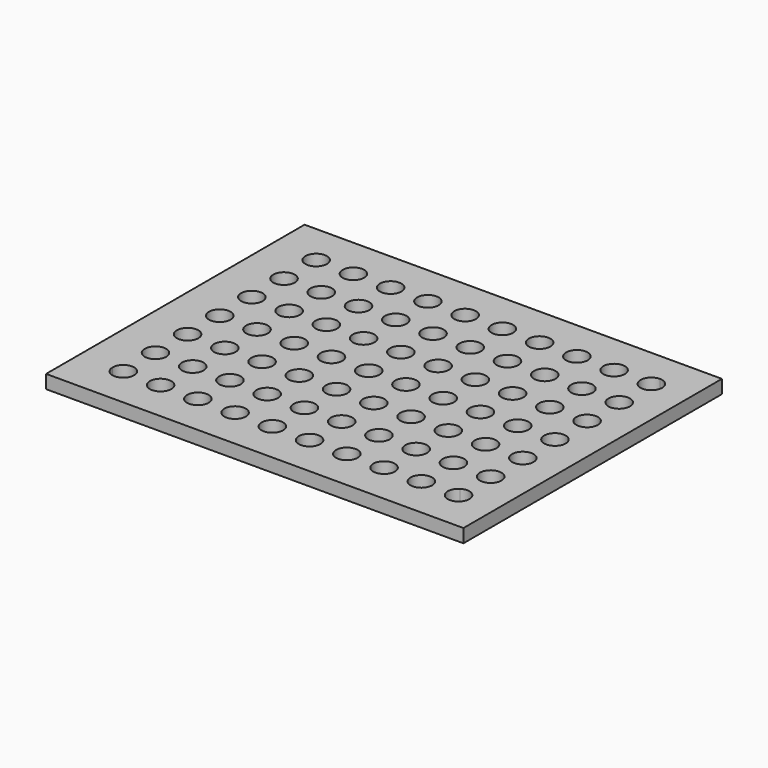
from build123d import *

# Parameters (mm, degrees)
F0_W     = 620
F0_H     = 480
F0_R     = 16
F1_DEPTH = 20


# Not quite as in the source:
# - ends of sketch curves that miss each other by under 0.0002 mm in the source are joined


with BuildPart() as f1:
    # F0 (on Top) → F1 (new body)
    with BuildSketch(Plane.XY):
        Rectangle(F0_W, F0_H)
        with BuildLine():
            ThreePointArc((-228, -179), (-228.000003125, -179.0099999941), (-228.0000125, -179.0199999844))
            ThreePointArc((-228.0000125, -179.0199999844), (-244.0050000002, -195.0199992187), (-259.999996875, -179.01))
            ThreePointArc((-259.999996875, -179.01), (-244.0050000002, -163.0000007813), (-228, -179))
        make_face(mode=Mode.SUBTRACT)
        with Locations((-188.67, -179.02)):
            Circle(F0_R, mode=Mode.SUBTRACT)
        with Locations((-133.34, -179.02)):
            Circle(F0_R, mode=Mode.SUBTRACT)
        with Locations((-78.01, -179.02)):
            Circle(F0_R, mode=Mode.SUBTRACT)
        with Locations((-22.68, -179.02)):
            Circle(F0_R, mode=Mode.SUBTRACT)
        with Locations((-244, -119.35)):
            Circle(F0_R, mode=Mode.SUBTRACT)
        with Locations((-188.67, -119.35)):
            Circle(F0_R, mode=Mode.SUBTRACT)
        with Locations((-244, -59.68)):
            Circle(F0_R, mode=Mode.SUBTRACT)
        with Locations((-244, -0.01)):
            Circle(F0_R, mode=Mode.SUBTRACT)
        with Locations((-188.67, -59.68)):
            Circle(F0_R, mode=Mode.SUBTRACT)
        with Locations((-188.67, -0.01)):
            Circle(F0_R, mode=Mode.SUBTRACT)
        with Locations((-133.34, -119.35)):
            Circle(F0_R, mode=Mode.SUBTRACT)
        with Locations((-78.01, -119.35)):
            Circle(F0_R, mode=Mode.SUBTRACT)
        with Locations((-22.68, -119.35)):
            Circle(F0_R, mode=Mode.SUBTRACT)
        with Locations((-133.34, -59.68)):
            Circle(F0_R, mode=Mode.SUBTRACT)
        with Locations((-78.01, -59.68)):
            Circle(F0_R, mode=Mode.SUBTRACT)
        with Locations((-133.34, -0.01)):
            Circle(F0_R, mode=Mode.SUBTRACT)
        with Locations((-78.01, -0.01)):
            Circle(F0_R, mode=Mode.SUBTRACT)
        with Locations((-22.68, -59.68)):
            Circle(F0_R, mode=Mode.SUBTRACT)
        with Locations((-22.68, -0.01)):
            Circle(F0_R, mode=Mode.SUBTRACT)
        with Locations((32.65, -179.02)):
            Circle(F0_R, mode=Mode.SUBTRACT)
        with Locations((87.98, -179.02)):
            Circle(F0_R, mode=Mode.SUBTRACT)
        with Locations((143.31, -179.02)):
            Circle(F0_R, mode=Mode.SUBTRACT)
        with Locations((198.64, -179.02)):
            Circle(F0_R, mode=Mode.SUBTRACT)
        with BuildLine():
            ThreePointArc((245.1098024941, -165.6972037411), (261.5417783017, -164.8889553878), (270, -179))
            ThreePointArc((270, -179), (268.1025380711, -186.5576729191), (262.8601975059, -192.3227962589))
            ThreePointArc((262.8601975059, -192.3227962589), (240.6571952906, -187.8952031396), (245.1098024941, -165.6972037411))
        make_face(mode=Mode.SUBTRACT)
        with Locations((32.65, -119.35)):
            Circle(F0_R, mode=Mode.SUBTRACT)
        with Locations((87.98, -119.35)):
            Circle(F0_R, mode=Mode.SUBTRACT)
        with Locations((143.31, -119.35)):
            Circle(F0_R, mode=Mode.SUBTRACT)
        with Locations((32.65, -59.68)):
            Circle(F0_R, mode=Mode.SUBTRACT)
        with Locations((32.65, -0.01)):
            Circle(F0_R, mode=Mode.SUBTRACT)
        with Locations((87.98, -59.68)):
            Circle(F0_R, mode=Mode.SUBTRACT)
        with Locations((143.31, -59.68)):
            Circle(F0_R, mode=Mode.SUBTRACT)
        with Locations((87.98, -0.01)):
            Circle(F0_R, mode=Mode.SUBTRACT)
        with Locations((143.31, -0.01)):
            Circle(F0_R, mode=Mode.SUBTRACT)
        with Locations((198.64, -119.35)):
            Circle(F0_R, mode=Mode.SUBTRACT)
        with Locations((253.97, -119.35)):
            Circle(F0_R, mode=Mode.SUBTRACT)
        with Locations((198.64, -59.68)):
            Circle(F0_R, mode=Mode.SUBTRACT)
        with Locations((198.64, -0.01)):
            Circle(F0_R, mode=Mode.SUBTRACT)
        with Locations((253.97, -59.68)):
            Circle(F0_R, mode=Mode.SUBTRACT)
        with Locations((253.97, -0.01)):
            Circle(F0_R, mode=Mode.SUBTRACT)
        with Locations((-244, 59.66)):
            Circle(F0_R, mode=Mode.SUBTRACT)
        with Locations((-188.67, 59.66)):
            Circle(F0_R, mode=Mode.SUBTRACT)
        with Locations((-244, 119.33)):
            Circle(F0_R, mode=Mode.SUBTRACT)
        with Locations((-188.67, 119.33)):
            Circle(F0_R, mode=Mode.SUBTRACT)
        with Locations((-133.34, 59.66)):
            Circle(F0_R, mode=Mode.SUBTRACT)
        with Locations((-78.01, 59.66)):
            Circle(F0_R, mode=Mode.SUBTRACT)
        with Locations((-22.68, 59.66)):
            Circle(F0_R, mode=Mode.SUBTRACT)
        with Locations((-133.34, 119.33)):
            Circle(F0_R, mode=Mode.SUBTRACT)
        with Locations((-78.01, 119.33)):
            Circle(F0_R, mode=Mode.SUBTRACT)
        with Locations((-22.68, 119.33)):
            Circle(F0_R, mode=Mode.SUBTRACT)
        with Locations((-244, 179)):
            Circle(F0_R, mode=Mode.SUBTRACT)
        with Locations((-188.67, 179)):
            Circle(F0_R, mode=Mode.SUBTRACT)
        with Locations((-133.34, 179)):
            Circle(F0_R, mode=Mode.SUBTRACT)
        with Locations((-78.01, 179)):
            Circle(F0_R, mode=Mode.SUBTRACT)
        with Locations((-22.68, 179)):
            Circle(F0_R, mode=Mode.SUBTRACT)
        with Locations((32.65, 59.66)):
            Circle(F0_R, mode=Mode.SUBTRACT)
        with Locations((87.98, 59.66)):
            Circle(F0_R, mode=Mode.SUBTRACT)
        with Locations((143.31, 59.66)):
            Circle(F0_R, mode=Mode.SUBTRACT)
        with Locations((32.65, 119.33)):
            Circle(F0_R, mode=Mode.SUBTRACT)
        with Locations((87.98, 119.33)):
            Circle(F0_R, mode=Mode.SUBTRACT)
        with Locations((143.31, 119.33)):
            Circle(F0_R, mode=Mode.SUBTRACT)
        with Locations((198.64, 59.66)):
            Circle(F0_R, mode=Mode.SUBTRACT)
        with Locations((253.97, 59.66)):
            Circle(F0_R, mode=Mode.SUBTRACT)
        with Locations((198.64, 119.33)):
            Circle(F0_R, mode=Mode.SUBTRACT)
        with Locations((253.97, 119.33)):
            Circle(F0_R, mode=Mode.SUBTRACT)
        with Locations((32.65, 179)):
            Circle(F0_R, mode=Mode.SUBTRACT)
        with Locations((87.98, 179)):
            Circle(F0_R, mode=Mode.SUBTRACT)
        with Locations((143.31, 179)):
            Circle(F0_R, mode=Mode.SUBTRACT)
        with Locations((198.64, 179)):
            Circle(F0_R, mode=Mode.SUBTRACT)
        with BuildLine():
            ThreePointArc((253.985, 194.9999929687), (265.3084039546, 190.3190105575), (270, 179))
            ThreePointArc((270, 179), (265.3084039546, 167.6809894425), (253.985, 163.0000070313))
            ThreePointArc((253.985, 163.0000070313), (237.97, 179), (253.985, 194.9999929687))
        make_face(mode=Mode.SUBTRACT)
    extrude(amount=F1_DEPTH)


solid = f1.part
